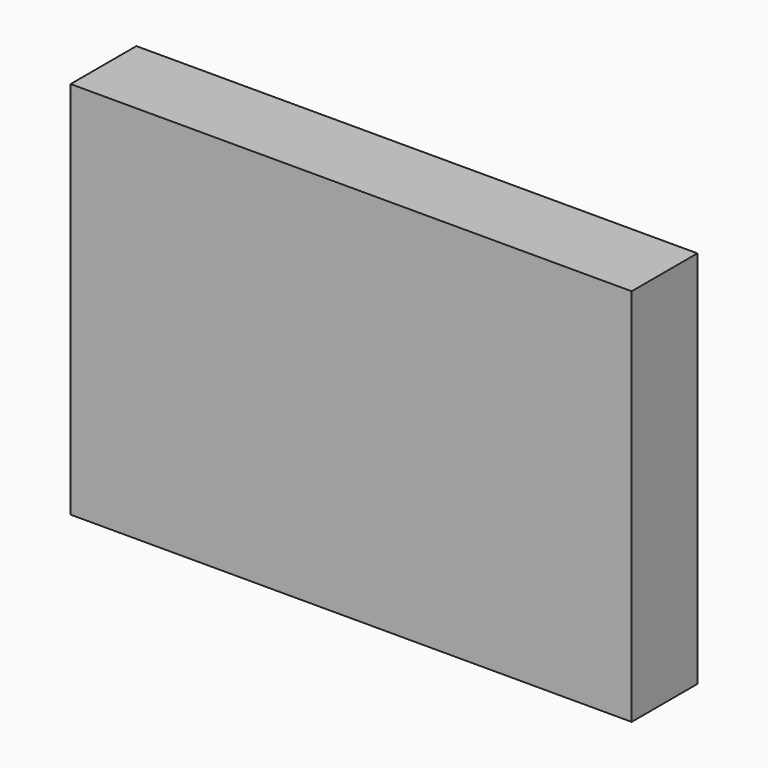
from build123d import *

# Parameters (mm, degrees)
F0_W     = 102.4124920368
F0_H     = 69.204211235
F1_DEPTH = 15


# Not quite as in the source:
# - the program builds the solid bodies; features that only make, move or delete a surface that nothing else refers to are left out


with BuildPart() as f1:
    # F0 (on Front) → F1 (new body)
    with BuildSketch(Plane.XZ):
        Rectangle(F0_W, F0_H)
    extrude(amount=F1_DEPTH)


solid = f1.part
